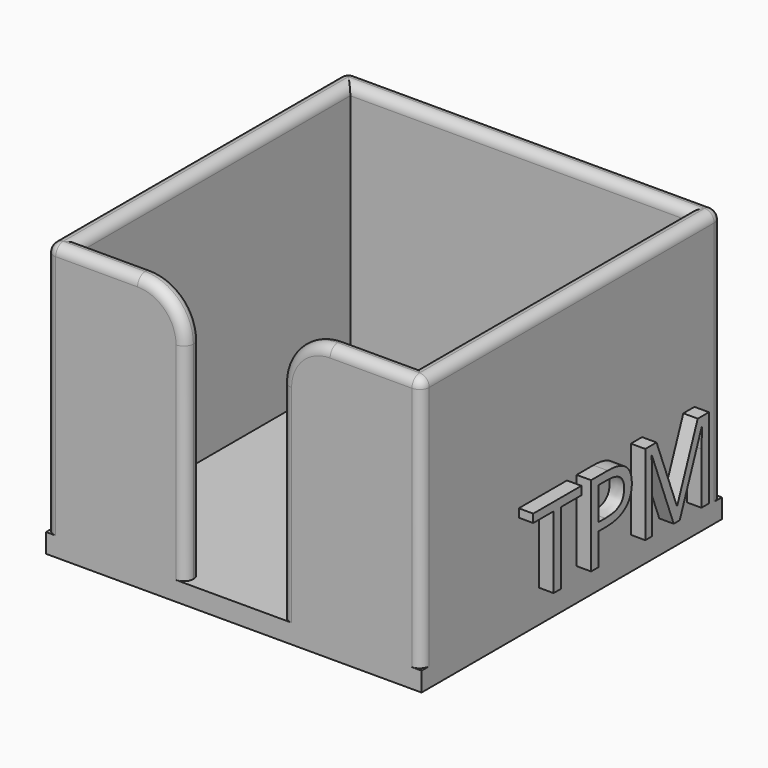
from build123d import *

# Parameters (mm, degrees)
F1_DEPTH     = 57
F2_R         = 10
F3_R         = 1.99999
F4_W         = 78
F4_H         = 78
F5_DEPTH     = 4
F6_TEXT_SIZE = 23.3762302539
F7_DEPTH     = 3
F8_TEXT_SIZE = 24.4356096826
F9_DEPTH     = 3


# Not quite as in the source:
# - a fillet or chamfer is up to 0.001 mm smaller than in the source, because OpenCascade refuses the exact size
# - Text() gives the source's letters only with a copy of the font that has no kerning and outlines rounded to 1/6400 em; it was checked with that copy


with BuildPart() as f1:
    # F0 (on Top) → F1 (new body)
    with BuildSketch(Plane.XY):
        Polygon((78, 0), (0, 0), (0, -78), (29, -78), (29, -74), (4, -74), (4, -4), (74, -4), (74, -74), (49, -74), (49, -78), (78, -78), align=None)
    extrude(amount=F1_DEPTH)

    # F2
    f2_edges = [f1.edges().sort_by_distance(p)[0] for p in [
        (29, -76, 57),
        (49, -76, 57),
    ]]
    fillet(f2_edges, radius=F2_R)

    # F3 (radius 2 in the source; OpenCascade refuses exactly that, so slightly less here)
    f3_edges = [f1.edges().sort_by_distance(p)[0] for p in [
        (9.5, -78, 57),
        (11.5, -74, 57),
        (4, -39, 57),
        (0, -39, 57),
        (39, -4, 57),
        (39, 0, 57),
        (78, -39, 57),
        (74, -39, 57),
        (66.5, -74, 57),
        (68.5, -78, 57),
        (0, -78, 28.5),
        (78, 0, 28.5),
        (78, -78, 28.5),
        (0, 0, 28.5),
    ]]
    fillet(f3_edges, radius=F3_R)

    # F4 (on Top) → F5 (join)
    with BuildSketch(Plane.XY):
        with Locations((39, -39)):
            Rectangle(F4_W, F4_H)
    extrude(amount=F5_DEPTH)

    # F6 (on face) → F7 (join)
    with BuildSketch(Plane.YZ.offset(78)):
        with Locations((-52.9555864632, 6.7513510585)):
            Text('TPM', F6_TEXT_SIZE, font='Open Sans', text_align=(TextAlign.LEFT, TextAlign.BOTTOM))
    extrude(amount=F7_DEPTH)

    # F8 (on face) → F9 (join)
    with BuildSketch(Plane(origin=(0, 0, 0), x_dir=(0, -1, 0), z_dir=(-1, 0, 0))):
        with Locations((6.4165443182, 7.5106434524)):
            Text('PMG', F8_TEXT_SIZE, font='Open Sans', text_align=(TextAlign.LEFT, TextAlign.BOTTOM))
    extrude(amount=F9_DEPTH)


solid = f1.part
